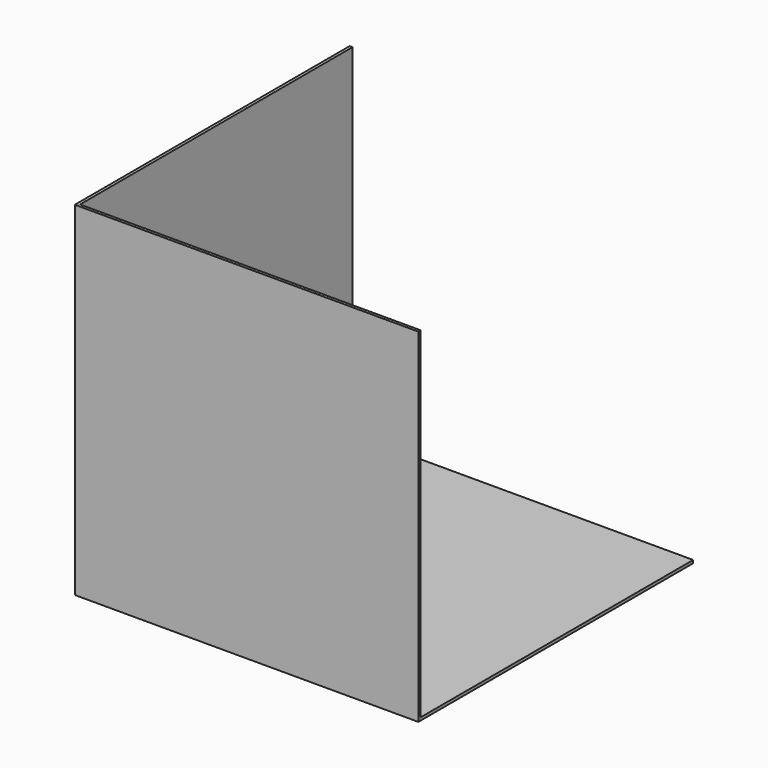
from build123d import *

# Parameters (mm, degrees)
F1_W      = 500
F1_H      = 500
F2_DEPTH  = 4.25
F3_W      = 500
F3_H      = 500
F4_DEPTH  = 4.25
F5_SIZE   = 4.24999
F5_2_SIZE = 4.24999
F6_W      = 495.75
F6_H      = 495.75
F7_DEPTH  = 4.25


# Not quite as in the source:
# - a fillet or chamfer is up to 0.001 mm smaller than in the source, because OpenCascade refuses the exact size


with BuildPart() as f2:
    # F1 (on Right) → F2 (new body)
    with BuildSketch(Plane.YZ):
        with Locations((250, 250)):
            Rectangle(F1_W, F1_H)
    extrude(amount=F2_DEPTH)

    # F5 (size 4.25 in the source; OpenCascade refuses exactly that, so slightly less here)
    f5_edges = [f2.edges().sort_by_distance(p)[0] for p in [
        (4.25, 0, 250),
    ]]
    chamfer(f5_edges, length=F5_SIZE)


with BuildPart() as f4:
    # F3 (on Front) → F4 (new body)
    with BuildSketch(Plane.XZ):
        with Locations((250, 250)):
            Rectangle(F3_W, F3_H)
    extrude(amount=-F4_DEPTH)

    # F5#2 (size 4.25 in the source; OpenCascade refuses exactly that, so slightly less here)
    f5_2_edges = [f4.edges().sort_by_distance(p)[0] for p in [
        (0, 4.25, 250),
    ]]
    chamfer(f5_2_edges, length=F5_2_SIZE)


with BuildPart() as f7:
    # F6 (on face) → F7 (new body)
    with BuildSketch(Plane(origin=(0, 0, 0), x_dir=(1, 0, 0), z_dir=(0, 0, -1))):
        with Locations((252.125, -252.125)):
            Rectangle(F6_W, F6_H)
    extrude(amount=-F7_DEPTH)


solid = Compound([f2.part, f4.part, f7.part])
